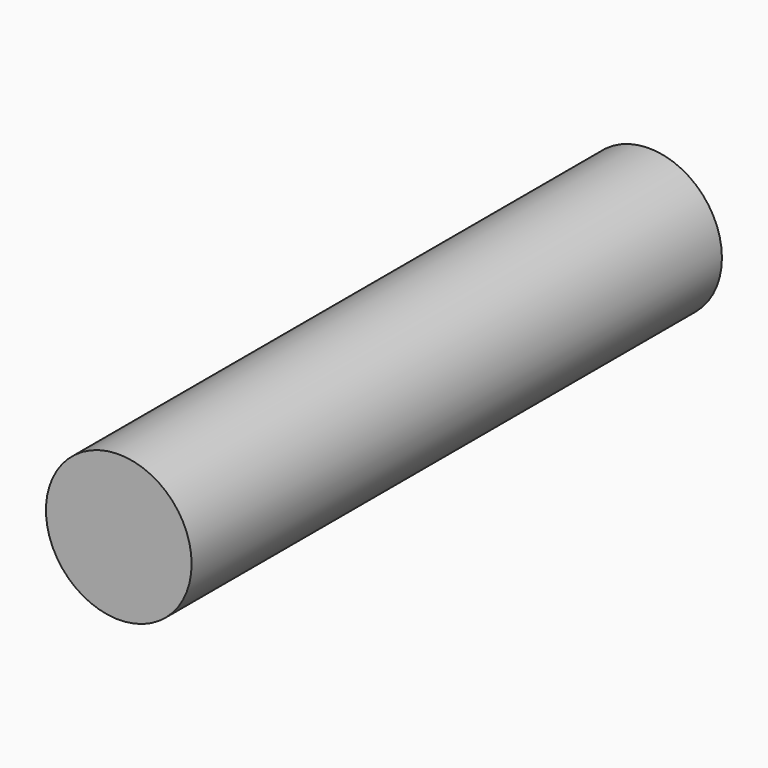
from build123d import *

# Parameters (mm, degrees)
F0_R     = 13.9551824708
F1_DEPTH = 127


# Not quite as in the source:
# - the program builds the solid bodies; features that only make, move or delete a surface that nothing else refers to are left out


with BuildPart() as f1:
    # F0 (on Front) → F1 (new body)
    with BuildSketch(Plane.XZ):
        Circle(F0_R)
    extrude(amount=F1_DEPTH)


solid = f1.part
